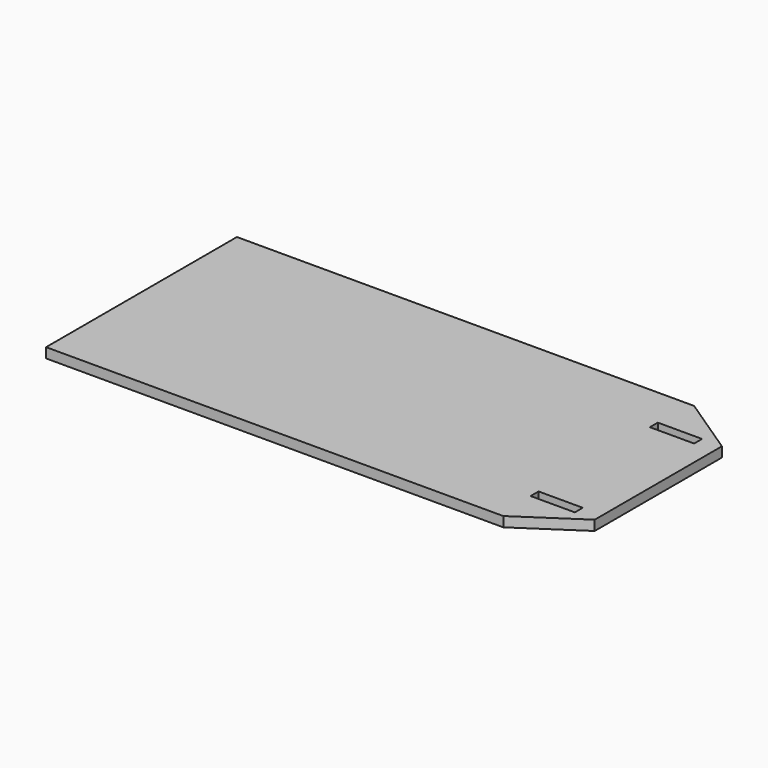
from build123d import *

# Parameters (mm, degrees)
F0_W     = 127
F0_H     = 76.2
F1_DEPTH = 3.175
F2_W     = 14.131395125
F2_H     = 3.175
F3_DEPTH = 25.4


# Not quite as in the source:
# - a length typed as a fraction of an inch, garbled in the dataset ("3 / 203.2 mm" for 3/8 in), is restored


with BuildPart() as f1:
    # F0 (on Top) → F1 (new body)
    with BuildSketch(Plane.XY):
        Polygon((84.1955885406, 47.9249996081), (65.1455885406, 47.9249996081), (65.1455885406, -28.2750003919), (84.1955885406, -28.2750003919), (103.2455885406, -15.5750003919), (103.2455885406, 35.2249996081), align=None)
        with Locations((1.6455885406, 9.8249996081)):
            Rectangle(F0_W, F0_H)
    extrude(amount=F1_DEPTH)

    # F2 (on face) → F3 (cut)
    with BuildSketch(Plane.XY.offset(3.175)):
        with Locations((89.8298909781, 33.6374996081)):
            Rectangle(F2_W, F2_H)
        with Locations((89.8298909781, -13.9875003919)):
            Rectangle(F2_W, F2_H)
    extrude(amount=-F3_DEPTH, mode=Mode.SUBTRACT)


solid = f1.part
